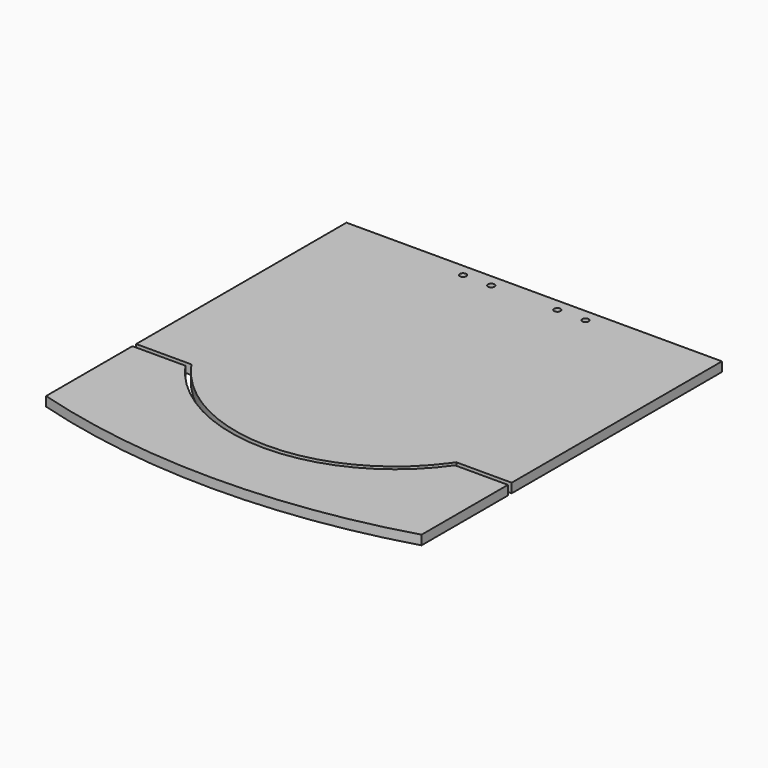
from build123d import *

# Parameters (mm, degrees)
F0_W      = 508
F0_H      = 508
F1_DEPTH  = 12.7
F3_DEPTH  = 25.4
F5_DEPTH  = 12.7
F6_R      = 1.5875
F7_DEPTH  = 11.43
F8_R      = 1.5875
F9_DEPTH  = 11.43
F10_R     = 4.365625
F11_DEPTH = 12.7


with BuildPart() as f1:
    # F0 (on Top) → F1 (new body)
    with BuildSketch(Plane.XY):
        Rectangle(F0_W, F0_H)
    extrude(amount=F1_DEPTH)

    # F2 (on face) → F3 (cut)
    with BuildSketch(Plane.XY.offset(12.7)):
        with BuildLine():
            ThreePointArc((174.5961339778, -107.95), (0, -196.85), (-174.5961339778, -107.95))
            ThreePointArc((-174.5961339778, -107.95), (-176.8480584357, -104.7949604446), (-179.0429766844, -101.6))
            Line((-179.0429766844, -101.6), (-186.6511184001, -101.6))
            Line((-186.6511184001, -101.6), (-254, -101.6))
            Line((-254, -101.6), (-254, -107.95))
            Line((-254, -107.95), (-182.3898640276, -107.95))
            ThreePointArc((-182.3898640276, -107.95), (0, -203.2), (182.3898640276, -107.95))
            Line((182.3898640276, -107.95), (254, -107.95))
            Line((254, -107.95), (254, -101.6))
            Line((254, -101.6), (186.6511184001, -101.6))
            Line((186.6511184001, -101.6), (179.0429766844, -101.6))
            ThreePointArc((179.0429766844, -101.6), (176.8480584357, -104.7949604446), (174.5961339778, -107.95))
        make_face()
    extrude(amount=-F3_DEPTH, mode=Mode.SUBTRACT)

    # F4 (on face) → F5 (join, through all)
    with BuildSketch(Plane.XY.offset(12.7)):
        with BuildLine():
            Line((254, -254), (-254, -254))
            ThreePointArc((-254, -254), (0, -290.5782934508), (254, -254))
        make_face()
    extrude(amount=-F5_DEPTH)

    # F6 (on face) → F7 (cut)
    with BuildSketch(Plane(origin=(0, 0, 0), x_dir=(1, 0, 0), z_dir=(0, 0, -1))):
        with Locations((203.2, -203.2)):
            Circle(F6_R)
        with Locations((-203.2, -203.2)):
            Circle(F6_R)
        with Locations((-203.2, 50.8)):
            Circle(F6_R)
        with Locations((203.2, 50.8)):
            Circle(F6_R)
        with Locations((0, 158.75)):
            Circle(F6_R)
    extrude(amount=-F7_DEPTH, mode=Mode.SUBTRACT)

    # F8 (on face) → F9 (cut)
    with BuildSketch(Plane(origin=(0, 0, 0), x_dir=(1, 0, 0), z_dir=(0, 0, -1))):
        with Locations((-165.1, 222.25)):
            Circle(F8_R)
        with Locations((165.1, 222.25)):
            Circle(F8_R)
    extrude(amount=-F9_DEPTH, mode=Mode.SUBTRACT)

    # F10 (on face) → F11 (cut, through all)
    with BuildSketch(Plane.XY.offset(12.7)):
        with Locations((44.704, 237.236)):
            Circle(F10_R)
        with Locations((82.804, 237.236)):
            Circle(F10_R)
        with Locations((-44.704, 237.236)):
            Circle(F10_R)
        with Locations((-82.804, 237.236)):
            Circle(F10_R)
    extrude(amount=-F11_DEPTH, mode=Mode.SUBTRACT)


solid = f1.part
